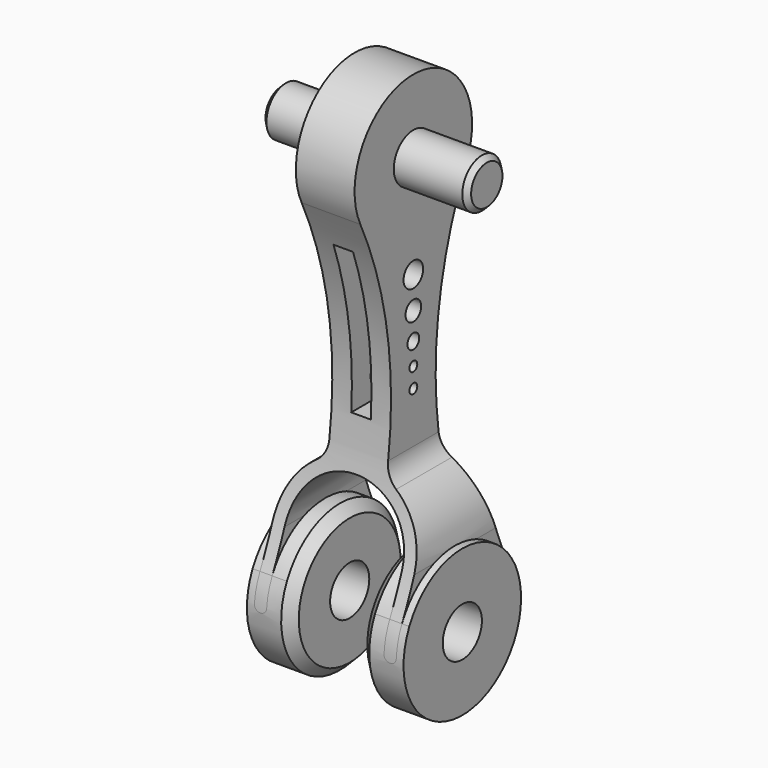
from build123d import *

# Parameters (mm, degrees)
F1_DEPTH  = 22.225
F3_R      = 19.05
F4_DEPTH  = 20.32
F2_R      = 6.35
F6_DEPTH  = 38.1
F5_W      = 17.78
F5_H      = 38.1
F7_DEPTH  = 19.05
F8_SIZE   = 2.54
F10_DEPTH = 7.62
F11_R     = 6.35
F12_DEPTH = 26.67
F13_SIZE  = 1.27
F15_DEPTH = 38.1
F16_W     = 5.08
F16_H     = 40.64
F17_DEPTH = 25.4
F18_R     = 6.35
F19_DEPTH = 19.05
F20_R     = 1.905
F20_R_2   = 1.27
F20_R_3   = 2.54
F20_R_4   = 3.175
F21_DEPTH = 12.7
F22_SIZE  = 1.27


with BuildPart() as f1:
    # F0 (on Front) → F1 (new body, symmetric)
    with BuildSketch(Plane.XZ):
        with BuildLine():
            Line((7.62, 0), (-7.62, 0))
            Line((-7.62, 0), (-7.62, -24.5142909701))
            Line((-7.62, -24.5142909701), (-7.62, -27.8114224211))
            ThreePointArc((-7.62, -27.8114224211), (-8.3544623748, -30.77591853), (-10.3879487179, -33.0546474413))
            ThreePointArc((-10.3879487179, -33.0546474413), (-16.2850591132, -39.6629612843), (-18.415, -48.26))
            Line((-18.415, -48.26), (-18.415, -64.516))
            ThreePointArc((-18.415, -64.516), (-17.9686307345, -65.5936307345), (-16.891, -66.04))
            Line((-16.891, -66.04), (-16.764, -66.04))
            ThreePointArc((-16.764, -66.04), (-15.6863692655, -65.5936307345), (-15.24, -64.516))
            Line((-15.24, -64.516), (-15.24, -48.26))
            ThreePointArc((-15.24, -48.26), (0, -33.02), (15.24, -48.26))
            Line((15.24, -48.26), (15.24, -65.0540764831))
            ThreePointArc((15.24, -65.0540764831), (15.6863692655, -66.1317072176), (16.764, -66.5780764831))
            Line((16.764, -66.5780764831), (16.891, -66.5780764831))
            ThreePointArc((16.891, -66.5780764831), (17.9686307345, -66.1317072176), (18.415, -65.0540764831))
            Line((18.415, -65.0540764831), (18.415, -48.26))
            ThreePointArc((18.415, -48.26), (16.2850591132, -39.6629612843), (10.3879487179, -33.0546474413))
            ThreePointArc((10.3879487179, -33.0546474413), (8.3544623748, -30.77591853), (7.62, -27.8114224211))
            Line((7.62, -27.8114224211), (7.62, -24.5142909701))
            Line((7.62, -24.5142909701), (7.62, 0))
        make_face()
    extrude(amount=F1_DEPTH, both=True)

    # F3 (on Right) → F4 (join, symmetric)
    with BuildSketch(Plane.YZ):
        with Locations((0, -66.04)):
            Circle(F3_R)
    extrude(amount=F4_DEPTH, both=True)

    # F2 (on Right) → F6 (cut, symmetric)
    with BuildSketch(Plane.YZ):
        with Locations((0, -66.04)):
            Circle(F2_R)
    extrude(amount=F6_DEPTH, both=True, mode=Mode.SUBTRACT)

    # F5 (on Front) → F7 (cut, symmetric)
    with BuildSketch(Plane.XZ):
        with Locations((0, -66.04)):
            Rectangle(F5_W, F5_H)
    extrude(amount=F7_DEPTH, both=True, mode=Mode.SUBTRACT)

    # F8
    f8_edges = [f1.edges().sort_by_distance(p)[0] for p in [
        (-8.89, -19.05, -66.04),
        (8.89, -19.05, -66.04),
    ]]
    chamfer(f8_edges, length=F8_SIZE)

    # F9 (on Right) → F10 (join, symmetric)
    with BuildSketch(Plane.YZ):
        with BuildLine():
            Line((19.0499954742, -0.0131314098), (19.0499954742, 38.0868685902))
            ThreePointArc((19.0499954742, 38.0868685902), (0, 57.15), (-19.0499954742, 38.0868685902))
            Line((-19.0499954742, 38.0868685902), (-19.0499954742, -0.0131314098))
            Line((-19.0499954742, -0.0131314098), (19.0499954742, -0.0131314098))
        make_face()
    extrude(amount=F10_DEPTH, both=True)

    # F11 (on Right) → F12 (join)
    with BuildSketch(Plane.YZ):
        with Locations((0, 38.1)):
            Circle(F11_R)
    extrude(amount=F12_DEPTH)

    # F13
    f13_edges = [f1.edges().sort_by_distance(p)[0] for p in [
        (26.67, -6.35, 38.1),
    ]]
    chamfer(f13_edges, length=F13_SIZE)

    # F14 (on Right) → F15 (intersect, symmetric)
    with BuildSketch(Plane.YZ):
        with BuildLine():
            ThreePointArc((17.184531987, -57.8184210526), (7.235369251, -13.97), (17.184531987, 29.8784210526))
            ThreePointArc((17.184531987, 29.8784210526), (0, 57.15), (-17.184531987, 29.8784210526))
            ThreePointArc((-17.184531987, 29.8784210526), (-7.235369251, -13.97), (-17.184531987, -57.8184210526))
            ThreePointArc((-17.184531987, -57.8184210526), (0, -85.09), (17.184531987, -57.8184210526))
        make_face()
    extrude(amount=F15_DEPTH, both=True, mode=Mode.INTERSECT)

    # F16 (on Front) → F17 (cut, symmetric)
    with BuildSketch(Plane.XZ):
        Rectangle(F16_W, F16_H)
    extrude(amount=F17_DEPTH, both=True, mode=Mode.SUBTRACT)

    # F18 (on face) → F19 (join)
    with BuildSketch(Plane(origin=(-7.62, 0, 0), x_dir=(0, -1, 0), z_dir=(-1, 0, 0))):
        with Locations((0, 38.1)):
            Circle(F18_R)
    extrude(amount=F19_DEPTH)

    # F20 (on Right) → F21 (cut, symmetric)
    with BuildSketch(Plane.YZ):
        with Locations((0, -3.81)):
            Circle(F20_R)
        with Locations((0, -9.525)):
            Circle(F20_R_2)
        with Locations((0, -14.605)):
            Circle(F20_R_2)
        with Locations((0, 3.175)):
            Circle(F20_R_3)
        with Locations((0, 11.43)):
            Circle(F20_R_4)
    extrude(amount=F21_DEPTH, both=True, mode=Mode.SUBTRACT)

    # F22
    f22_edges = [f1.edges().sort_by_distance(p)[0] for p in [
        (-26.67, 6.35, 38.1),
    ]]
    chamfer(f22_edges, length=F22_SIZE)


with BuildPart() as f1_1:
    # F24: moved
    add(f1.part.moved(Location((0, 0, -38.1))))


solid = f1_1.part
